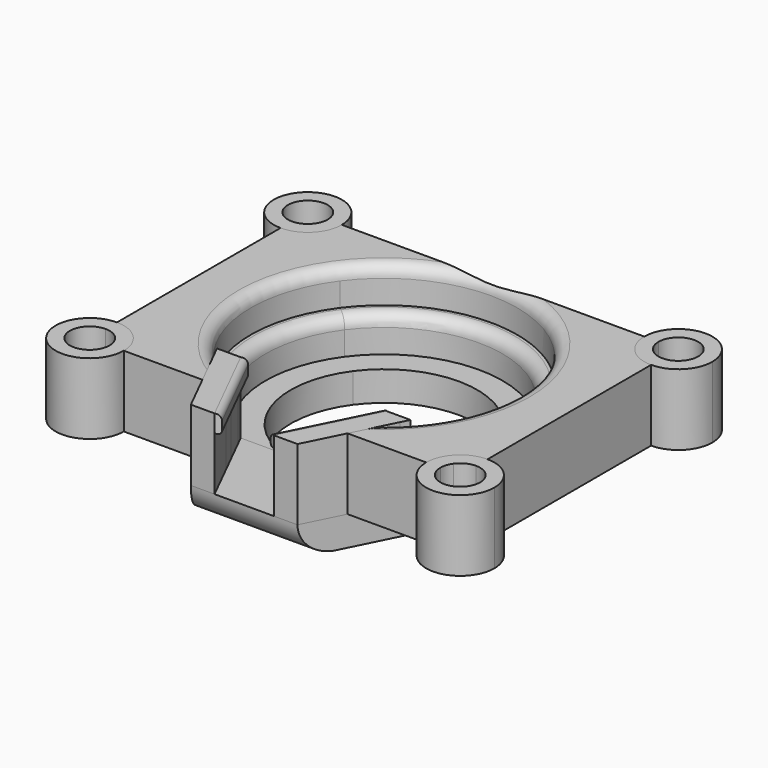
from build123d import *

# Parameters (mm, degrees)
F1_DEPTH    = 12
F2_DEPTH    = 5
F3_DEPTH    = 5
F4_DEPTH    = 6
F5_DEPTH    = 12
F6_R        = 2
F7_T2_ANGLE = 335.3184227228
F8_DEPTH    = 5
F9_DEPTH    = 12
F10_W       = 16.404
F10_H       = 2
F11_DEPTH   = 1
F12_R       = 0.99999
F13_R       = 0.5
F14_W       = 16.404
F14_H       = 3
F15_DEPTH   = 1
F16_R       = 0.99999
F17_R       = 0.5
F18_R       = 4.99999
F19_R       = 1.25


# Not quite as in the source:
# - a fillet or chamfer that OpenCascade refuses, or shapes differently, is made with other operations: its cross-section is extruded or revolved along the edge and cut away or added
# - a fillet or chamfer is up to 0.001 mm smaller than in the source, because OpenCascade refuses the exact size


with BuildPart() as f1:
    # F0 (on Top) → F1 (new body)
    with BuildSketch(Plane.XY):
        with BuildLine():
            Line((-31.2666631574, -19.65), (-31.2666631574, -17.25))
            ThreePointArc((-31.2666631574, -17.25), (-35.3325271492, -27.0658639918), (-25.5166631574, -23))
            Line((-25.5166631574, -23), (-27.9166631574, -23))
            ThreePointArc((-27.9166631574, -23), (-33.6354708744, -25.368807717), (-31.2666631574, -19.65))
        make_face()
        with BuildLine():
            ThreePointArc((-25.5166631574, -23), (-27.2007991656, -18.9341360082), (-31.2666631574, -17.25))
            Line((-31.2666631574, -17.25), (-31.2666631574, -19.65))
            ThreePointArc((-31.2666631574, -19.65), (-28.8978554405, -20.631192283), (-27.9166631574, -23))
            Line((-27.9166631574, -23), (-25.5166631574, -23))
        make_face()
    extrude(amount=F1_DEPTH)


with BuildPart() as f1b:
    # F0 (on Top) → F1, piece 2 (new body)
    with BuildSketch(Plane.XY):
        with BuildLine():
            ThreePointArc((37.0166631574, 23), (31.2666631574, 28.75), (25.5166631574, 23))
            Line((25.5166631574, 23), (27.9166631574, 23))
            ThreePointArc((27.9166631574, 23), (31.2666631574, 26.35), (34.6166631574, 23))
            ThreePointArc((34.6166631574, 23), (33.6354708744, 20.631192283), (31.2666631574, 19.65))
            Line((31.2666631574, 19.65), (31.2666631574, 17.25))
            ThreePointArc((31.2666631574, 17.25), (35.3325271492, 18.9341360082), (37.0166631574, 23))
        make_face()
        with BuildLine():
            Line((27.9166631574, 23), (25.5166631574, 23))
            ThreePointArc((25.5166631574, 23), (27.2007991656, 18.9341360082), (31.2666631574, 17.25))
            Line((31.2666631574, 17.25), (31.2666631574, 19.65))
            ThreePointArc((31.2666631574, 19.65), (28.8978554405, 20.631192283), (27.9166631574, 23))
        make_face()
    extrude(amount=F1_DEPTH)


with BuildPart() as f1c:
    # F0 (on Top) → F1, piece 3 (new body)
    with BuildSketch(Plane.XY):
        with BuildLine():
            Line((-27.9166631574, 23), (-25.5166631574, 23))
            ThreePointArc((-25.5166631574, 23), (-35.3325271492, 27.0658639918), (-31.2666631574, 17.25))
            Line((-31.2666631574, 17.25), (-31.2666631574, 19.65))
            ThreePointArc((-31.2666631574, 19.65), (-33.6354708744, 25.368807717), (-27.9166631574, 23))
        make_face()
        with BuildLine():
            Line((-31.2666631574, 19.65), (-31.2666631574, 17.25))
            ThreePointArc((-31.2666631574, 17.25), (-28.6713626614, 17.8690239393), (-26.6348632565, 19.5928120572))
            Line((-26.6348632565, 19.5928120572), (-28.5681362586, 21.0149426768))
            ThreePointArc((-28.5681362586, 21.0149426768), (-29.7546185206, 20.0106487298), (-31.2666631574, 19.65))
        make_face()
        with BuildLine():
            ThreePointArc((-26.6348632565, 19.5928120572), (-25.8033606109, 21.2070066133), (-25.5166631574, 23))
            Line((-25.5166631574, 23), (-27.9166631574, 23))
            ThreePointArc((-27.9166631574, 23), (-28.0836955868, 21.9553864617), (-28.5681362586, 21.0149426768))
            Line((-28.5681362586, 21.0149426768), (-26.6348632565, 19.5928120572))
        make_face()
    extrude(amount=F1_DEPTH)


with BuildPart() as f1d:
    # F0 (on Top) → F1, piece 4 (new body)
    with BuildSketch(Plane.XY):
        with BuildLine():
            ThreePointArc((37.0166631574, -23), (35.3325271492, -18.9341360082), (31.2666631574, -17.25))
            Line((31.2666631574, -17.25), (31.2666631574, -19.65))
            ThreePointArc((31.2666631574, -19.65), (33.6354708744, -20.631192283), (34.6166631574, -23))
            ThreePointArc((34.6166631574, -23), (31.2666631574, -26.35), (27.9166631574, -23))
            Line((27.9166631574, -23), (25.5166631574, -23))
            ThreePointArc((25.5166631574, -23), (31.2666631574, -28.75), (37.0166631574, -23))
        make_face()
        with BuildLine():
            Line((31.2666631574, -19.65), (31.2666631574, -17.25))
            ThreePointArc((31.2666631574, -17.25), (28.6713626614, -17.8690239393), (26.6348632565, -19.5928120572))
            Line((26.6348632565, -19.5928120572), (28.5681362586, -21.0149426768))
            ThreePointArc((28.5681362586, -21.0149426768), (29.7546185206, -20.0106487298), (31.2666631574, -19.65))
        make_face()
        with BuildLine():
            Line((28.5681362586, -21.0149426768), (26.6348632565, -19.5928120572))
            ThreePointArc((26.6348632565, -19.5928120572), (25.8033606109, -21.2070066133), (25.5166631574, -23))
            Line((25.5166631574, -23), (27.9166631574, -23))
            ThreePointArc((27.9166631574, -23), (28.0836955868, -21.9553864617), (28.5681362586, -21.0149426768))
        make_face()
    extrude(amount=F1_DEPTH)


with BuildPart() as f2:
    # F0 (on Top) → F2 (new body)
    with BuildSketch(Plane.XY):
        with BuildLine():
            ThreePointArc((5.3256589686, -14.8222756873), (2.7029296999, -15.5163356189), (0, -15.75))
            Line((0, -15.75), (0, -20))
            ThreePointArc((0, -20), (6.081235767, -19.0530462537), (11.5866066348, -16.3018571546))
            Line((11.5866066348, -16.3018571546), (12.325, -14.8222756873))
            Line((12.325, -14.8222756873), (5.3256589686, -14.8222756873))
        make_face()
        with BuildLine():
            ThreePointArc((13.4275888919, -14.8222756873), (14.8436269969, -13.4039821537), (16.1106083511, -11.8510884967))
            Line((16.1106083511, -11.8510884967), (12.6871040765, -9.3327321912))
            ThreePointArc((12.6871040765, -9.3327321912), (9.415342802, -12.6259185773), (5.3256589686, -14.8222756873))
            Line((5.3256589686, -14.8222756873), (12.325, -14.8222756873))
            Line((12.325, -14.8222756873), (13.4275888919, -14.8222756873))
        make_face()
        with BuildLine():
            ThreePointArc((11.5866066348, -16.3018571546), (12.5289578494, -15.5892660253), (13.4275888919, -14.8222756873))
            Line((13.4275888919, -14.8222756873), (12.325, -14.8222756873))
            Line((12.325, -14.8222756873), (11.5866066348, -16.3018571546))
        make_face()
        with BuildLine():
            ThreePointArc((20, 0), (6.2364987364, 19.0027914663), (-16.1106083511, 11.8510884967))
            Line((-16.1106083511, 11.8510884967), (-12.6871040765, 9.3327321912))
            ThreePointArc((-12.6871040765, 9.3327321912), (4.9112427549, 14.9646982797), (15.75, 0))
            ThreePointArc((15.75, 0), (14.9646982797, -4.9112427549), (12.6871040765, -9.3327321912))
            Line((12.6871040765, -9.3327321912), (16.1106083511, -11.8510884967))
            ThreePointArc((16.1106083511, -11.8510884967), (19.0027914663, -6.2364987364), (20, 0))
        make_face()
        with BuildLine():
            Line((-12.6871040765, 9.3327321912), (-16.1106083511, 11.8510884967))
            ThreePointArc((-16.1106083511, 11.8510884967), (-19.8995819884, -2.0016584836), (-13.4275888919, -14.8222756873))
            Line((-13.4275888919, -14.8222756873), (-12.325, -14.8222756873))
            Line((-12.325, -14.8222756873), (-5.3256589686, -14.8222756873))
            ThreePointArc((-5.3256589686, -14.8222756873), (-15.0658889393, -4.591458425), (-12.6871040765, 9.3327321912))
        make_face()
        with BuildLine():
            ThreePointArc((0, -15.75), (-2.7029296999, -15.5163356189), (-5.3256589686, -14.8222756873))
            Line((-5.3256589686, -14.8222756873), (-12.325, -14.8222756873))
            Line((-12.325, -14.8222756873), (-11.5866066348, -16.3018571546))
            ThreePointArc((-11.5866066348, -16.3018571546), (-6.081235767, -19.0530462537), (0, -20))
            Line((0, -20), (0, -15.75))
        make_face()
        with BuildLine():
            Line((-12.325, -14.8222756873), (-13.4275888919, -14.8222756873))
            ThreePointArc((-13.4275888919, -14.8222756873), (-12.5289578494, -15.5892660253), (-11.5866066348, -16.3018571546))
            Line((-11.5866066348, -16.3018571546), (-12.325, -14.8222756873))
        make_face()
    extrude(amount=-F2_DEPTH)

    # F0 (on Top) → F3 (join)
    with BuildSketch(Plane.XY):
        with BuildLine():
            Line((-16.325, -14.8222756873), (-15.6588908732, -16.1570150901))
            ThreePointArc((-15.6588908732, -16.1570150901), (-12.7824589423, -18.5164452147), (-9.5565572057, -20.3696395249))
            Line((-9.5565572057, -20.3696395249), (-11.5866066348, -16.3018571546))
            ThreePointArc((-11.5866066348, -16.3018571546), (-12.5289578494, -15.5892660253), (-13.4275888919, -14.8222756873))
            Line((-13.4275888919, -14.8222756873), (-16.325, -14.8222756873))
        make_face()
        with BuildLine():
            Line((-16.1106083511, 11.8510884967), (-18.124434395, 13.3324745588))
            ThreePointArc((-18.124434395, 13.3324745588), (-22.4217699231, -1.8746289013), (-15.6588908732, -16.1570150901))
            Line((-15.6588908732, -16.1570150901), (-16.325, -14.8222756873))
            Line((-16.325, -14.8222756873), (-13.4275888919, -14.8222756873))
            ThreePointArc((-13.4275888919, -14.8222756873), (-19.8995819884, -2.0016584836), (-16.1106083511, 11.8510884967))
        make_face()
        with BuildLine():
            ThreePointArc((22.5, 0), (7.0160610784, 21.3781403996), (-18.124434395, 13.3324745588))
            Line((-18.124434395, 13.3324745588), (-16.1106083511, 11.8510884967))
            ThreePointArc((-16.1106083511, 11.8510884967), (6.2364987364, 19.0027914663), (20, 0))
            ThreePointArc((20, 0), (19.0027914663, -6.2364987364), (16.1106083511, -11.8510884967))
            Line((16.1106083511, -11.8510884967), (18.124434395, -13.3324745588))
            ThreePointArc((18.124434395, -13.3324745588), (21.3781403996, -7.0160610784), (22.5, 0))
        make_face()
        with BuildLine():
            ThreePointArc((15.6588908732, -16.1570150901), (16.950598038, -14.7961895822), (18.124434395, -13.3324745588))
            Line((18.124434395, -13.3324745588), (16.1106083511, -11.8510884967))
            ThreePointArc((16.1106083511, -11.8510884967), (14.8436269969, -13.4039821537), (13.4275888919, -14.8222756873))
            Line((13.4275888919, -14.8222756873), (16.325, -14.8222756873))
            Line((16.325, -14.8222756873), (15.6588908732, -16.1570150901))
        make_face()
        with BuildLine():
            ThreePointArc((9.5565572057, -20.3696395249), (12.7824589423, -18.5164452147), (15.6588908732, -16.1570150901))
            Line((15.6588908732, -16.1570150901), (16.325, -14.8222756873))
            Line((16.325, -14.8222756873), (13.4275888919, -14.8222756873))
            ThreePointArc((13.4275888919, -14.8222756873), (12.5289578494, -15.5892660253), (11.5866066348, -16.3018571546))
            Line((11.5866066348, -16.3018571546), (9.5565572057, -20.3696395249))
        make_face()
        with BuildLine():
            Line((0, -20), (0, -22.5))
            ThreePointArc((0, -22.5), (4.8955648647, -21.9609527265), (9.5565572057, -20.3696395249))
            Line((9.5565572057, -20.3696395249), (11.5866066348, -16.3018571546))
            ThreePointArc((11.5866066348, -16.3018571546), (6.081235767, -19.0530462537), (0, -20))
        make_face()
        with BuildLine():
            Line((-11.5866066348, -16.3018571546), (-9.5565572057, -20.3696395249))
            ThreePointArc((-9.5565572057, -20.3696395249), (-4.8955648647, -21.9609527265), (0, -22.5))
            Line((0, -22.5), (0, -20))
            ThreePointArc((0, -20), (-6.081235767, -19.0530462537), (-11.5866066348, -16.3018571546))
        make_face()
    extrude(amount=-F3_DEPTH)

    # F0 (on Top) → F4 (join)
    with BuildSketch(Plane.XY):
        with BuildLine():
            Line((-16.1106083511, 11.8510884967), (-18.124434395, 13.3324745588))
            ThreePointArc((-18.124434395, 13.3324745588), (-22.4217699231, -1.8746289013), (-15.6588908732, -16.1570150901))
            Line((-15.6588908732, -16.1570150901), (-16.325, -14.8222756873))
            Line((-16.325, -14.8222756873), (-13.4275888919, -14.8222756873))
            ThreePointArc((-13.4275888919, -14.8222756873), (-19.8995819884, -2.0016584836), (-16.1106083511, 11.8510884967))
        make_face()
        with BuildLine():
            Line((-16.325, -14.8222756873), (-15.6588908732, -16.1570150901))
            ThreePointArc((-15.6588908732, -16.1570150901), (-12.7824589423, -18.5164452147), (-9.5565572057, -20.3696395249))
            Line((-9.5565572057, -20.3696395249), (-11.5866066348, -16.3018571546))
            ThreePointArc((-11.5866066348, -16.3018571546), (-12.5289578494, -15.5892660253), (-13.4275888919, -14.8222756873))
            Line((-13.4275888919, -14.8222756873), (-16.325, -14.8222756873))
        make_face()
        with BuildLine():
            ThreePointArc((9.5565572057, -20.3696395249), (12.7824589423, -18.5164452147), (15.6588908732, -16.1570150901))
            Line((15.6588908732, -16.1570150901), (16.325, -14.8222756873))
            Line((16.325, -14.8222756873), (13.4275888919, -14.8222756873))
            ThreePointArc((13.4275888919, -14.8222756873), (12.5289578494, -15.5892660253), (11.5866066348, -16.3018571546))
            Line((11.5866066348, -16.3018571546), (9.5565572057, -20.3696395249))
        make_face()
        with BuildLine():
            ThreePointArc((15.6588908732, -16.1570150901), (16.950598038, -14.7961895822), (18.124434395, -13.3324745588))
            Line((18.124434395, -13.3324745588), (16.1106083511, -11.8510884967))
            ThreePointArc((16.1106083511, -11.8510884967), (14.8436269969, -13.4039821537), (13.4275888919, -14.8222756873))
            Line((13.4275888919, -14.8222756873), (16.325, -14.8222756873))
            Line((16.325, -14.8222756873), (15.6588908732, -16.1570150901))
        make_face()
        with BuildLine():
            ThreePointArc((22.5, 0), (7.0160610784, 21.3781403996), (-18.124434395, 13.3324745588))
            Line((-18.124434395, 13.3324745588), (-16.1106083511, 11.8510884967))
            ThreePointArc((-16.1106083511, 11.8510884967), (6.2364987364, 19.0027914663), (20, 0))
            ThreePointArc((20, 0), (19.0027914663, -6.2364987364), (16.1106083511, -11.8510884967))
            Line((16.1106083511, -11.8510884967), (18.124434395, -13.3324745588))
            ThreePointArc((18.124434395, -13.3324745588), (21.3781403996, -7.0160610784), (22.5, 0))
        make_face()
    extrude(amount=F4_DEPTH)

    # F6
    f6_edges = [f2.edges().sort_by_distance(p)[0] for p in [
        (0, 20, 6),
    ]]
    fillet(f6_edges, radius=F6_R)

    # F19
    f19_edges = [f2.edges().sort_by_distance(p)[0] for p in [
        (9.556557, 20.36964, -5),
    ]]
    fillet(f19_edges, radius=F19_R)


with BuildPart() as f5:
    # F0 (on Top) → F5 (new body)
    with BuildSketch(Plane.XY):
        with BuildLine():
            ThreePointArc((-26.6348632565, 19.5928120572), (-28.6713626614, 17.8690239393), (-31.2666631574, 17.25))
            Line((-31.2666631574, 17.25), (-31.2666631574, -17.25))
            ThreePointArc((-31.2666631574, -17.25), (-27.2007991656, -18.9341360082), (-25.5166631574, -23))
            Line((-25.5166631574, -23), (-12.2438611726, -23))
            Line((-12.2438611726, -23), (-15.6588908732, -16.1570150901))
            ThreePointArc((-15.6588908732, -16.1570150901), (-22.4217699231, -1.8746289013), (-18.124434395, 13.3324745588))
            Line((-18.124434395, 13.3324745588), (-26.6348632565, 19.5928120572))
        make_face()
        with BuildLine():
            Line((25.5166631574, 23), (-25.5166631574, 23))
            ThreePointArc((-25.5166631574, 23), (-25.8033606109, 21.2070066133), (-26.6348632565, 19.5928120572))
            Line((-26.6348632565, 19.5928120572), (-18.124434395, 13.3324745588))
            ThreePointArc((-18.124434395, 13.3324745588), (7.0160610784, 21.3781403996), (22.5, 0))
            ThreePointArc((22.5, 0), (21.3781403996, -7.0160610784), (18.124434395, -13.3324745588))
            Line((18.124434395, -13.3324745588), (26.6348632565, -19.5928120572))
            ThreePointArc((26.6348632565, -19.5928120572), (28.6713626614, -17.8690239393), (31.2666631574, -17.25))
            Line((31.2666631574, -17.25), (31.2666631574, 17.25))
            ThreePointArc((31.2666631574, 17.25), (27.2007991656, 18.9341360082), (25.5166631574, 23))
        make_face()
        with BuildLine():
            Line((26.6348632565, -19.5928120572), (18.124434395, -13.3324745588))
            ThreePointArc((18.124434395, -13.3324745588), (16.950598038, -14.7961895822), (15.6588908732, -16.1570150901))
            Line((15.6588908732, -16.1570150901), (12.2438611726, -23))
            Line((12.2438611726, -23), (25.5166631574, -23))
            ThreePointArc((25.5166631574, -23), (25.8033606109, -21.2070066133), (26.6348632565, -19.5928120572))
        make_face()
        with BuildLine():
            ThreePointArc((-9.5565572057, -20.3696395249), (-12.7824589423, -18.5164452147), (-15.6588908732, -16.1570150901))
            Line((-15.6588908732, -16.1570150901), (-12.2438611726, -23))
            Line((-12.2438611726, -23), (-8.2438611726, -23))
            Line((-8.2438611726, -23), (-9.5565572057, -20.3696395249))
        make_face()
        with BuildLine():
            Line((12.2438611726, -23), (15.6588908732, -16.1570150901))
            ThreePointArc((15.6588908732, -16.1570150901), (12.7824589423, -18.5164452147), (9.5565572057, -20.3696395249))
            Line((9.5565572057, -20.3696395249), (8.2438611726, -23))
            Line((8.2438611726, -23), (12.2438611726, -23))
        make_face()
    extrude(amount=F5_DEPTH)

    # F7: fillet of radius 2 on 1 edges, made by hand

    # F7_s1 → F7_t2 (revolve, cut)
    with BuildSketch(Plane(origin=(0, 0, 0), x_dir=(0, 0, 1), z_dir=(0.9768936714, -0.2137258871, 0))):
        with BuildLine():
            ThreePointArc((10, 22.5), (11.4142135624, 23.0857864376), (12, 24.5))
            Line((12, 24.5), (12, 22.5))
            Line((12, 22.5), (10, 22.5))
        make_face()
    revolve(axis=Axis((0, 0, 12), (0, 0, -1)), revolution_arc=F7_T2_ANGLE, mode=Mode.SUBTRACT)


with BuildPart() as f8:
    # F0 (on Top) → F8 (new body)
    with BuildSketch(Plane.XY):
        Polygon((9, -29.5), (12.2438611726, -23), (8.2438611726, -23), (5, -29.5), align=None)
        with BuildLine():
            Line((12.2438611726, -23), (15.6588908732, -16.1570150901))
            ThreePointArc((15.6588908732, -16.1570150901), (12.7824589423, -18.5164452147), (9.5565572057, -20.3696395249))
            Line((9.5565572057, -20.3696395249), (8.2438611726, -23))
            Line((8.2438611726, -23), (12.2438611726, -23))
        make_face()
        with BuildLine():
            ThreePointArc((9.5565572057, -20.3696395249), (12.7824589423, -18.5164452147), (15.6588908732, -16.1570150901))
            Line((15.6588908732, -16.1570150901), (16.325, -14.8222756873))
            Line((16.325, -14.8222756873), (13.4275888919, -14.8222756873))
            ThreePointArc((13.4275888919, -14.8222756873), (12.5289578494, -15.5892660253), (11.5866066348, -16.3018571546))
            Line((11.5866066348, -16.3018571546), (9.5565572057, -20.3696395249))
        make_face()
        with BuildLine():
            ThreePointArc((11.5866066348, -16.3018571546), (12.5289578494, -15.5892660253), (13.4275888919, -14.8222756873))
            Line((13.4275888919, -14.8222756873), (12.325, -14.8222756873))
            Line((12.325, -14.8222756873), (11.5866066348, -16.3018571546))
        make_face()
        with BuildLine():
            Line((-12.325, -14.8222756873), (-13.4275888919, -14.8222756873))
            ThreePointArc((-13.4275888919, -14.8222756873), (-12.5289578494, -15.5892660253), (-11.5866066348, -16.3018571546))
            Line((-11.5866066348, -16.3018571546), (-12.325, -14.8222756873))
        make_face()
        with BuildLine():
            Line((-16.325, -14.8222756873), (-15.6588908732, -16.1570150901))
            ThreePointArc((-15.6588908732, -16.1570150901), (-12.7824589423, -18.5164452147), (-9.5565572057, -20.3696395249))
            Line((-9.5565572057, -20.3696395249), (-11.5866066348, -16.3018571546))
            ThreePointArc((-11.5866066348, -16.3018571546), (-12.5289578494, -15.5892660253), (-13.4275888919, -14.8222756873))
            Line((-13.4275888919, -14.8222756873), (-16.325, -14.8222756873))
        make_face()
        with BuildLine():
            ThreePointArc((-9.5565572057, -20.3696395249), (-12.7824589423, -18.5164452147), (-15.6588908732, -16.1570150901))
            Line((-15.6588908732, -16.1570150901), (-12.2438611726, -23))
            Line((-12.2438611726, -23), (-8.2438611726, -23))
            Line((-8.2438611726, -23), (-9.5565572057, -20.3696395249))
        make_face()
        Polygon((-8.2438611726, -23), (-12.2438611726, -23), (-9, -29.5), (-5, -29.5), align=None)
        Polygon((0, -23), (-8.2438611726, -23), (-5, -29.5), (0, -29.5), align=None)
        with BuildLine():
            ThreePointArc((0, -22.5), (-4.8955648647, -21.9609527265), (-9.5565572057, -20.3696395249))
            Line((-9.5565572057, -20.3696395249), (-8.2438611726, -23))
            Line((-8.2438611726, -23), (0, -23))
            Line((0, -23), (0, -22.5))
        make_face()
        Polygon((8.2438611726, -23), (0, -23), (0, -29.5), (5, -29.5), align=None)
        with BuildLine():
            ThreePointArc((9.5565572057, -20.3696395249), (4.8955648647, -21.9609527265), (0, -22.5))
            Line((0, -22.5), (0, -23))
            Line((0, -23), (8.2438611726, -23))
            Line((8.2438611726, -23), (9.5565572057, -20.3696395249))
        make_face()
        with BuildLine():
            Line((0, -20), (0, -22.5))
            ThreePointArc((0, -22.5), (4.8955648647, -21.9609527265), (9.5565572057, -20.3696395249))
            Line((9.5565572057, -20.3696395249), (11.5866066348, -16.3018571546))
            ThreePointArc((11.5866066348, -16.3018571546), (6.081235767, -19.0530462537), (0, -20))
        make_face()
        with BuildLine():
            Line((-11.5866066348, -16.3018571546), (-9.5565572057, -20.3696395249))
            ThreePointArc((-9.5565572057, -20.3696395249), (-4.8955648647, -21.9609527265), (0, -22.5))
            Line((0, -22.5), (0, -20))
            ThreePointArc((0, -20), (-6.081235767, -19.0530462537), (-11.5866066348, -16.3018571546))
        make_face()
        with BuildLine():
            ThreePointArc((0, -15.75), (-2.7029296999, -15.5163356189), (-5.3256589686, -14.8222756873))
            Line((-5.3256589686, -14.8222756873), (-12.325, -14.8222756873))
            Line((-12.325, -14.8222756873), (-11.5866066348, -16.3018571546))
            ThreePointArc((-11.5866066348, -16.3018571546), (-6.081235767, -19.0530462537), (0, -20))
            Line((0, -20), (0, -15.75))
        make_face()
        with BuildLine():
            ThreePointArc((5.3256589686, -14.8222756873), (2.7029296999, -15.5163356189), (0, -15.75))
            Line((0, -15.75), (0, -20))
            ThreePointArc((0, -20), (6.081235767, -19.0530462537), (11.5866066348, -16.3018571546))
            Line((11.5866066348, -16.3018571546), (12.325, -14.8222756873))
            Line((12.325, -14.8222756873), (5.3256589686, -14.8222756873))
        make_face()
    extrude(amount=-F8_DEPTH)

    # F18 (radius 5 in the source; OpenCascade refuses exactly that, so slightly less here)
    f18_edges = [f8.edges().sort_by_distance(p)[0] for p in [
        (0, -29.5, -5),
    ]]
    fillet(f18_edges, radius=F18_R)


with BuildPart() as f9:
    # F0 (on Top) → F9 (new body)
    with BuildSketch(Plane.XY):
        with BuildLine():
            Line((-16.325, -14.8222756873), (-15.6588908732, -16.1570150901))
            ThreePointArc((-15.6588908732, -16.1570150901), (-12.7824589423, -18.5164452147), (-9.5565572057, -20.3696395249))
            Line((-9.5565572057, -20.3696395249), (-11.5866066348, -16.3018571546))
            ThreePointArc((-11.5866066348, -16.3018571546), (-12.5289578494, -15.5892660253), (-13.4275888919, -14.8222756873))
            Line((-13.4275888919, -14.8222756873), (-16.325, -14.8222756873))
        make_face()
        with BuildLine():
            Line((-12.325, -14.8222756873), (-13.4275888919, -14.8222756873))
            ThreePointArc((-13.4275888919, -14.8222756873), (-12.5289578494, -15.5892660253), (-11.5866066348, -16.3018571546))
            Line((-11.5866066348, -16.3018571546), (-12.325, -14.8222756873))
        make_face()
        with BuildLine():
            ThreePointArc((-9.5565572057, -20.3696395249), (-12.7824589423, -18.5164452147), (-15.6588908732, -16.1570150901))
            Line((-15.6588908732, -16.1570150901), (-12.2438611726, -23))
            Line((-12.2438611726, -23), (-8.2438611726, -23))
            Line((-8.2438611726, -23), (-9.5565572057, -20.3696395249))
        make_face()
        Polygon((-8.2438611726, -23), (-12.2438611726, -23), (-9, -29.5), (-5, -29.5), align=None)
    extrude(amount=F9_DEPTH)


with BuildPart() as f9b:
    # F0 (on Top) → F9, piece 2 (new body)
    with BuildSketch(Plane.XY):
        Polygon((9, -29.5), (12.2438611726, -23), (8.2438611726, -23), (5, -29.5), align=None)
        with BuildLine():
            Line((12.2438611726, -23), (15.6588908732, -16.1570150901))
            ThreePointArc((15.6588908732, -16.1570150901), (12.7824589423, -18.5164452147), (9.5565572057, -20.3696395249))
            Line((9.5565572057, -20.3696395249), (8.2438611726, -23))
            Line((8.2438611726, -23), (12.2438611726, -23))
        make_face()
        with BuildLine():
            ThreePointArc((9.5565572057, -20.3696395249), (12.7824589423, -18.5164452147), (15.6588908732, -16.1570150901))
            Line((15.6588908732, -16.1570150901), (16.325, -14.8222756873))
            Line((16.325, -14.8222756873), (13.4275888919, -14.8222756873))
            ThreePointArc((13.4275888919, -14.8222756873), (12.5289578494, -15.5892660253), (11.5866066348, -16.3018571546))
            Line((11.5866066348, -16.3018571546), (9.5565572057, -20.3696395249))
        make_face()
        with BuildLine():
            ThreePointArc((11.5866066348, -16.3018571546), (12.5289578494, -15.5892660253), (13.4275888919, -14.8222756873))
            Line((13.4275888919, -14.8222756873), (12.325, -14.8222756873))
            Line((12.325, -14.8222756873), (11.5866066348, -16.3018571546))
        make_face()
    extrude(amount=F9_DEPTH)


with BuildPart() as f11:
    # F10 (on face) → F11 (new body)
    with BuildSketch(Plane(origin=(15.7896298905, -7.8799026664, 0), x_dir=(-0.4465374299, -0.8947649544, 0), z_dir=(-0.8947649544, 0.4465374299, 0))):
        with Locations((15.9608790066, 11)):
            Rectangle(F10_W, F10_H)
    extrude(amount=F11_DEPTH)

    # F12 (radius 1 in the source; OpenCascade refuses exactly that, so slightly less here)
    f12_edges = [f11.edges().sort_by_distance(p)[0] for p in [
        (7.767735, -21.7146, 12),
    ]]
    fillet(f12_edges, radius=F12_R)

    # F13
    f13_edges = [f11.edges().sort_by_distance(p)[0] for p in [
        (7.767735, -21.7146, 10),
    ]]
    fillet(f13_edges, radius=F13_R)


with BuildPart() as f15:
    # F14 (on face) → F15 (new body)
    with BuildSketch(Plane(origin=(-15.7896298905, -7.8799026664, 0), x_dir=(-0.4465374299, 0.8947649544, 0), z_dir=(0.8947649544, 0.4465374299, 0))):
        with Locations((-15.9608790066, 10.5)):
            Rectangle(F14_W, F14_H)
    extrude(amount=F15_DEPTH)

    # F16 (radius 1 in the source; OpenCascade refuses exactly that, so slightly less here)
    f16_edges = [f15.edges().sort_by_distance(p)[0] for p in [
        (-7.767735, -21.7146, 12),
    ]]
    fillet(f16_edges, radius=F16_R)

    # F17
    f17_edges = [f15.edges().sort_by_distance(p)[0] for p in [
        (-7.767735, -21.7146, 9),
    ]]
    fillet(f17_edges, radius=F17_R)


solid = Compound([f1.part, f1b.part, f1c.part, f1d.part, f2.part, f5.part, f8.part, f9.part, f9b.part, f11.part, f15.part])
